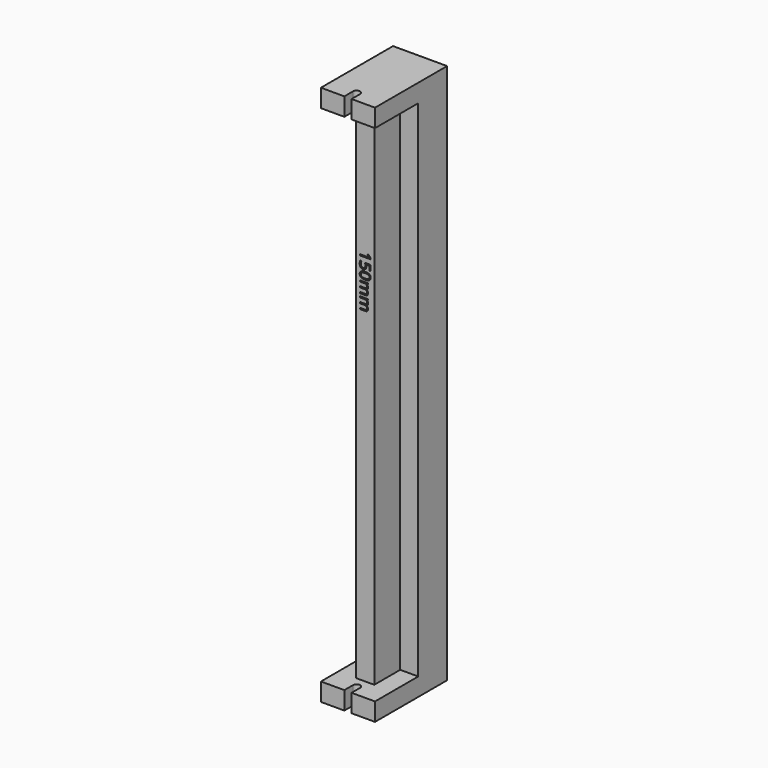
from build123d import *

# Parameters (mm, degrees)
F0_W         = 15
F0_H         = 25
F1_DEPTH     = 150
F2_W         = 15
F2_H         = 140
F3_DEPTH     = 5
F5_W         = 5
F5_H         = 140
F6_DEPTH     = 6
F8_DEPTH     = 150.001
F9_TEXT_SIZE = 4.1666666667
F10_DEPTH    = 1


# Not quite as in the source:
# - Text() gives the source's letters only with a copy of the font that has no kerning and outlines rounded to 1/6400 em; it was checked with that copy


with BuildPart() as f1:
    # F0 (on Top) → F1 (new body)
    with BuildSketch(Plane.XY):
        Rectangle(F0_W, F0_H)
    extrude(amount=F1_DEPTH)

    # F2 (on face) → F3 (cut)
    with BuildSketch(Plane.YZ.offset(7.5)):
        with Locations((-5, 75)):
            Rectangle(F2_W, F2_H)
    extrude(amount=-F3_DEPTH, mode=Mode.SUBTRACT)

    # F4: F1 across plane


with BuildPart() as f1_1:
    add(f1.part)
    add(f1.part.mirror(Plane.YZ), mode=Mode.INTERSECT)

    # F5 (on face) → F6 (cut)
    with BuildSketch(Plane.XZ.offset(12.5)):
        with Locations((0, 75)):
            Rectangle(F5_W, F5_H)
    extrude(amount=-F6_DEPTH, mode=Mode.SUBTRACT)

    # F7 (on face) → F8 (cut, through all)
    with BuildSketch(Plane.XY.offset(150)):
        with BuildLine():
            Line((-1, -9.5), (-1, -12.5))
            Line((-1, -12.5), (1, -12.5))
            Line((1, -12.5), (1, -9.5))
            ThreePointArc((1, -9.5), (0, -8.5), (-1, -9.5))
        make_face()
    extrude(amount=-F8_DEPTH, mode=Mode.SUBTRACT)

    # F9 (on face) → F10 (cut)
    with BuildSketch(Plane.XZ.offset(6.5)):
        with Locations(Location((-1.5, 110.0047871064), (0, 0, -90))):
            Text('150mm', F9_TEXT_SIZE, font='Open Sans', text_align=(TextAlign.LEFT, TextAlign.BOTTOM))
    extrude(amount=-F10_DEPTH, mode=Mode.SUBTRACT)


solid = f1_1.part
